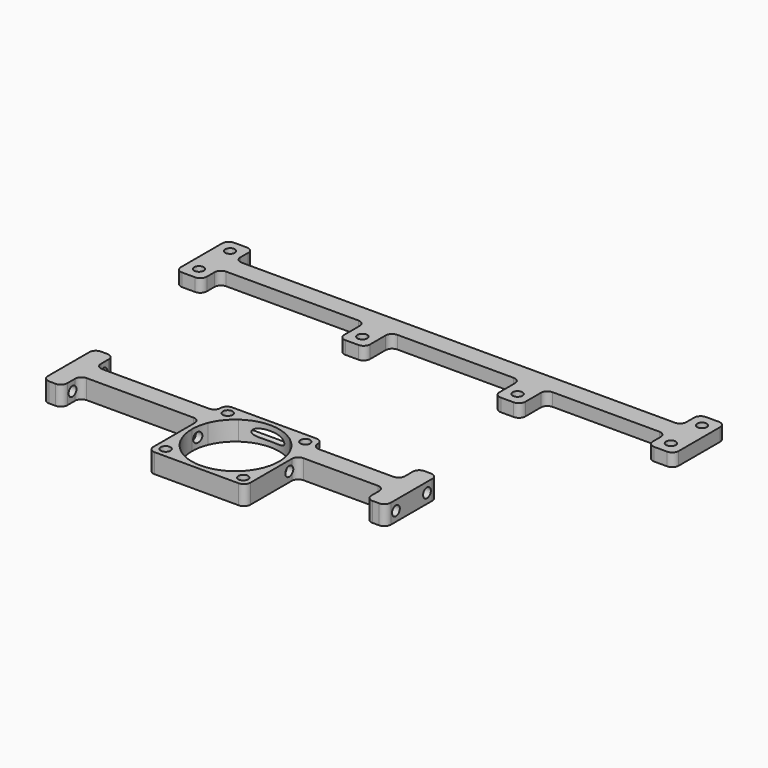
from build123d import *

# Parameters (mm, degrees)
F0_R     = 1.5
F0_W     = 8
F0_H     = 10
F1_DEPTH = 4
F6_R     = 2
F0_W_2   = 37
F0_H_2   = 6
F0_W_3   = 27
F2_DEPTH = 6
F3_R     = 1.99999
F3_2_R   = 1.99999
F4_R     = 1.5
F5_DEPTH = 118.8957548568


# Not quite as in the source:
# - a fillet or chamfer is up to 0.001 mm smaller than in the source, because OpenCascade refuses the exact size
# - a feature names something its author has since deleted; it is built from what else it names


with BuildPart() as f1:
    # F0 (on Top) → F1 (new body)
    with BuildSketch(Plane.XY):
        Polygon((-62.8947548568, -4), (-62.8947548568, 3), (-62.8947548568, 9), (-62.8947548568, 16), (-70.8947548568, 16), (-70.8947548568, -4), align=None)
        with Locations((-66.8947548568, 0)):
            Circle(F0_R, mode=Mode.SUBTRACT)
        with Locations((-66.8947548568, 12)):
            Circle(F0_R, mode=Mode.SUBTRACT)
        with Locations((-14, -2)):
            Rectangle(F0_W, F0_H)
        with Locations((-14, -3)):
            Circle(F0_R, mode=Mode.SUBTRACT)
        with Locations((34, -2)):
            Rectangle(F0_W, F0_H)
        with Locations((34, -3)):
            Circle(F0_R, mode=Mode.SUBTRACT)
        Polygon((75, 9), (75, 3), (75, -4), (83, -4), (83, 16), (75, 16), align=None)
        with Locations((79, 0)):
            Circle(F0_R, mode=Mode.SUBTRACT)
        with Locations((79, 12)):
            Circle(F0_R, mode=Mode.SUBTRACT)
        Polygon((-10, 3), (30, 3), (38, 3), (75, 3), (75, 9), (-62.8947548568, 9), (-62.8947548568, 3), (-18, 3), align=None)
    extrude(amount=F1_DEPTH)

    # F6
    f6_edges = [f1.edges().sort_by_distance(p)[0] for p in [
        (-70.894755, -4, 2),
        (-18, -7, 2),
        (-10, -7, 2),
        (-70.894755, 16, 2),
        (30, -7, 2),
        (38, -7, 2),
        (83, -4, 2),
        (83, 16, 2),
        (75, 16, 2),
        (-62.894755, 16, 2),
        (-62.894755, 3, 2),
        (-62.894755, 9, 2),
        (75, 3, 2),
        (75, 9, 2),
    ]]
    fillet(f6_edges, radius=F6_R)

    # F3#2 (radius 2 in the source; OpenCascade refuses exactly that, so slightly less here)
    f3_2_edges = [f1.edges().sort_by_distance(p)[0] for p in [
        (-62.894755, -4, 2),
        (-18, 3, 2),
        (-10, 3, 2),
        (30, 3, 2),
        (75, -4, 2),
        (38, 3, 2),
    ]]
    fillet(f3_2_edges, radius=F3_2_R)


with BuildPart() as f2:
    # F0 (on Top) → F2 (new body)
    with BuildSketch(Plane.XY):
        Polygon((-52, -64.51824072), (-52, -58.51824072), (-52, -51.51824072), (-58, -51.51824072), (-58, -71.51824072), (-52, -71.51824072), align=None)
        Polygon((48, -51.51824072), (42, -51.51824072), (42, -58.51824072), (42, -64.51824072), (42, -71.51824072), (48, -71.51824072), align=None)
        with BuildLine():
            Line((13.1180339887, -58.51824072), (15, -58.51824072))
            Line((15, -58.51824072), (15, -54.51824072))
            Line((15, -54.51824072), (-15, -54.51824072))
            Line((-15, -54.51824072), (-15, -58.51824072))
            Line((-15, -58.51824072), (-13.1180339887, -58.51824072))
            ThreePointArc((-13.1180339887, -58.51824072), (-12.5352331347, -56.1169821816), (-10.5, -57.51824072))
            ThreePointArc((-10.5, -57.51824072), (-10.5987414616, -58.0534738547), (-10.8819660113, -58.51824072))
            Line((-10.8819660113, -58.51824072), (-7.8262379212, -58.51824072))
            ThreePointArc((-7.8262379212, -58.51824072), (0, -56.01824072), (7.8262379212, -58.51824072))
            Line((7.8262379212, -58.51824072), (10.8819660113, -58.51824072))
            ThreePointArc((10.8819660113, -58.51824072), (11.4647668653, -56.1169821816), (13.5, -57.51824072))
            ThreePointArc((13.5, -57.51824072), (13.4012585384, -58.0534738547), (13.1180339887, -58.51824072))
        make_face()
        with Locations((-33.5, -61.51824072)):
            Rectangle(F0_W_2, F0_H_2)
        with BuildLine():
            Line((15, -84.51824072), (15, -69.51824072))
            Line((15, -69.51824072), (13.5, -69.51824072))
            ThreePointArc((13.5, -69.51824072), (0, -83.01824072), (-13.5, -69.51824072))
            Line((-13.5, -69.51824072), (-15, -69.51824072))
            Line((-15, -69.51824072), (-15, -84.51824072))
            Line((-15, -84.51824072), (15, -84.51824072))
        make_face()
        with Locations((-12, -81.51824072)):
            Circle(F0_R, mode=Mode.SUBTRACT)
        with Locations((12, -81.51824072)):
            Circle(F0_R, mode=Mode.SUBTRACT)
        with BuildLine():
            Line((-13.1180339887, -58.51824072), (-15, -58.51824072))
            Line((-15, -58.51824072), (-15, -64.51824072))
            Line((-15, -64.51824072), (-12.539936204, -64.51824072))
            ThreePointArc((-12.539936204, -64.51824072), (-10.615802472, -61.1782924063), (-7.8262379212, -58.51824072))
            Line((-7.8262379212, -58.51824072), (-10.8819660113, -58.51824072))
            ThreePointArc((-10.8819660113, -58.51824072), (-12, -59.01824072), (-13.1180339887, -58.51824072))
        make_face()
        with BuildLine():
            Line((15, -64.51824072), (15, -58.51824072))
            Line((15, -58.51824072), (13.1180339887, -58.51824072))
            ThreePointArc((13.1180339887, -58.51824072), (12, -59.01824072), (10.8819660113, -58.51824072))
            Line((10.8819660113, -58.51824072), (7.8262379212, -58.51824072))
            ThreePointArc((7.8262379212, -58.51824072), (10.615802472, -61.1782924063), (12.539936204, -64.51824072))
            Line((12.539936204, -64.51824072), (15, -64.51824072))
        make_face()
        with Locations((28.5, -61.51824072)):
            Rectangle(F0_W_3, F0_H_2)
        with BuildLine():
            Line((-15, -69.51824072), (-13.5, -69.51824072))
            ThreePointArc((-13.5, -69.51824072), (-13.257811636, -66.9725717268), (-12.539936204, -64.51824072))
            Line((-12.539936204, -64.51824072), (-15, -64.51824072))
            Line((-15, -64.51824072), (-15, -69.51824072))
        make_face()
        with BuildLine():
            Line((15, -69.51824072), (15, -64.51824072))
            Line((15, -64.51824072), (12.539936204, -64.51824072))
            ThreePointArc((12.539936204, -64.51824072), (13.257811636, -66.9725717268), (13.5, -69.51824072))
            Line((13.5, -69.51824072), (15, -69.51824072))
        make_face()
    extrude(amount=F2_DEPTH)

    # F3 (radius 2 in the source; OpenCascade refuses exactly that, so slightly less here)
    f3_edges = [f2.edges().sort_by_distance(p)[0] for p in [
        (-52, -58.518241, 3),
        (-52, -64.518241, 3),
        (-52, -71.518241, 3),
        (-58, -71.518241, 3),
        (42, -71.518241, 3),
        (48, -71.518241, 3),
        (48, -51.518241, 3),
        (-52, -51.518241, 3),
        (-58, -51.518241, 3),
        (42, -64.518241, 3),
        (42, -58.518241, 3),
        (42, -51.518241, 3),
        (-15, -54.518241, 3),
        (15, -54.518241, 3),
        (-15, -84.518241, 3),
        (15, -84.518241, 3),
        (15, -58.518241, 3),
        (15, -64.518241, 3),
        (-15, -64.518241, 3),
        (-15, -58.518241, 3),
    ]]
    fillet(f3_edges, radius=F3_R)

    # F4 (on face) → F5 (cut, through all)
    with BuildSketch(Plane.YZ.offset(48)):
        with Locations((-55.51824072, 3)):
            Circle(F4_R)
        with Locations((-67.51824072, 3)):
            Circle(F4_R)
    extrude(amount=-F5_DEPTH, mode=Mode.SUBTRACT)


solid = Compound([f1.part, f2.part])
